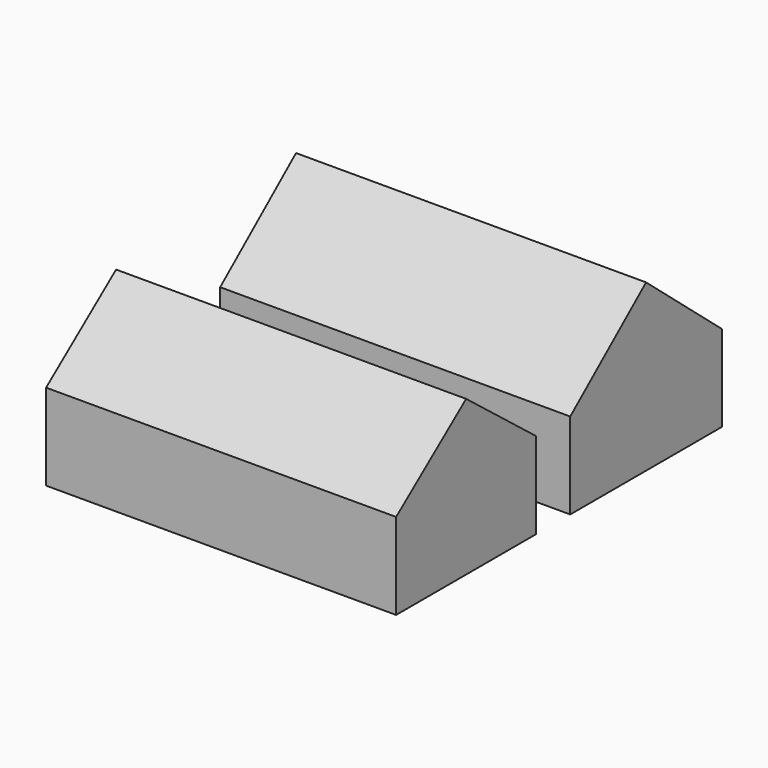
from build123d import *

# Parameters (mm, degrees)
F0_W     = 12000
F0_H     = 6500
F1_DEPTH = 2800
F3_DEPTH = 12000
F2_W     = 6000
F2_H     = 2958


# Not quite as in the source:
# - a feature names something its author has since deleted; it is built from what else it names


with BuildPart() as f1:
    # F0 (on Top) → F1 (new body)
    with BuildSketch(Plane.XY):
        Rectangle(F0_W, F0_H)
    extrude(amount=F1_DEPTH)

    # F2 (on face) → F3 (join)
    with BuildSketch(Plane(origin=(-6000, 0, 0), x_dir=(0, -1, 0), z_dir=(-1, 0, 0))):
        Polygon((-2254.2731399598, 3270), (-2814.3973284791, 2800), (-2254.2731399598, 2800), align=None)
        Polygon((-3250, 2956.6488747199), (-3250, 2800), (0, 5527.0738013262), (3250, 2800), (3250, 2956.6488747199), (3173.8782442282, 3020.5226119126), (0, 5683.722676046), (-3178.3420854061, 3016.7770044265), align=None)
        Polygon((2254.2731399598, 3270), (2254.2731399598, 2800), (2814.3973284791, 2800), align=None)
        Polygon((-2814.3973284791, 2800), (-3250, 2800), (-3250, 2570), (-2254.2731399598, 2570), (-2254.2731399598, 2800), align=None)
        Polygon((3250, 2570), (3250, 2800), (2814.3973284791, 2800), (2254.2731399598, 2800), (2254.2731399598, 2570), align=None)
        Polygon((-2254.2731399598, 2570), (-3250, 2570), (-3250, 2400), (3250, 2400), (3250, 2570), (2254.2731399598, 2570), align=None)
        Polygon((0, 5527.0738013262), (-3250, 2800), (-2814.3973284791, 2800), (-2254.2731399598, 3270), (-650, 4616.1450000479), (0, 5161.5597603131), (650, 4616.1450000479), (2254.2731399598, 3270), (2814.3973284791, 2800), (3250, 2800), align=None)
        Polygon((0, 5161.5597603131), (-650, 4616.1450000479), (650, 4616.1450000479), align=None)
        Polygon((-2254.2731399598, 3270), (-2254.2731399598, 2800), (2254.2731399598, 2800), (2254.2731399598, 3270), (650, 4616.1450000479), (-650, 4616.1450000479), align=None)
    extrude(amount=-F3_DEPTH)


with BuildPart() as f3:
    # F2 (on face) → F3, piece 2 (new body)
    with BuildSketch(Plane(origin=(-6000, 0, 0), x_dir=(0, -1, 0), z_dir=(-1, 0, 0))):
        Polygon((7709.972858429, 5301.8568795202), (4709.972858429, 2958), (10709.972858429, 2958), align=None)
        with Locations((7709.972858429, 1479)):
            Rectangle(F2_W, F2_H)
    extrude(amount=-F3_DEPTH)


solid = Compound([f1.part, f3.part])
